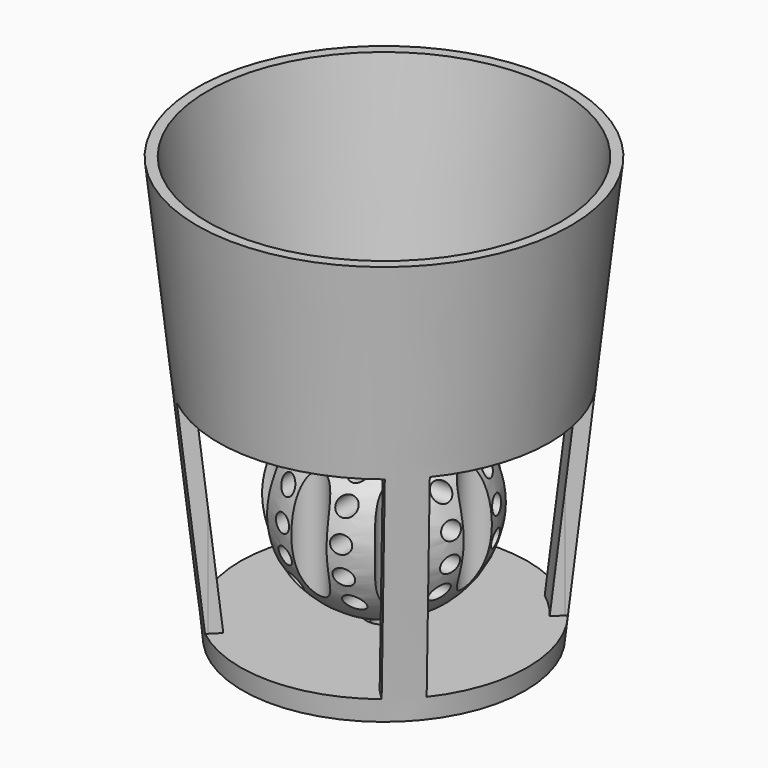
from build123d import *

# Parameters (mm, degrees)
F3_DEPTH      = 29
F4_R          = 2.5
F5_DEPTH      = 2
F5_DEPTH_BACK = 31
F8_R          = 2.5
F9_DEPTH      = 36.6
F10_R         = 1.25
F11_DEPTH     = 15
F12_R         = 1.25
F13_DEPTH     = 15


with BuildPart() as f1:
    # F0 (on Front) → F1 (revolve)
    with BuildSketch(Plane.XZ):
        Polygon((0, 3), (0, 0), (20, 0), (26.4482922192, 60), (25, 60), (22.3132115753, 35), (0, 35), (0, 32), (21.4275722125, 32), (18.3108976399, 3), align=None)
    revolve(axis=Axis((0, 0, 33.5), (0, 0, 1)))

    # F2 (on face) → F3 (cut)
    with BuildSketch(Plane.XY.offset(3)):
        with BuildLine():
            Line((12.2634482474, 15.7989821534), (15.6845353346, 19.2200692405))
            ThreePointArc((15.6845353346, 19.2200692405), (0, 24.8075736474), (-15.6845353346, 19.2200692405))
            Line((-15.6845353346, 19.2200692405), (-12.2634482474, 15.7989821534))
            Line((-12.2634482474, 15.7989821534), (-10.9417147938, 14.4772486998))
            ThreePointArc((-10.9417147938, 14.4772486998), (0, 18.1469516048), (10.9417147938, 14.4772486998))
            Line((10.9417147938, 14.4772486998), (12.2634482474, 15.7989821534))
        make_face()
        with BuildLine():
            Line((19.2200692405, 15.6845353346), (15.7989821534, 12.2634482474))
            Line((15.7989821534, 12.2634482474), (14.4772486998, 10.9417147938))
            ThreePointArc((14.4772486998, 10.9417147938), (18.1469516048, 0), (14.4772486998, -10.9417147938))
            Line((14.4772486998, -10.9417147938), (15.7989821534, -12.2634482474))
            Line((15.7989821534, -12.2634482474), (19.2200692405, -15.6845353346))
            ThreePointArc((19.2200692405, -15.6845353346), (24.8075736474, 0), (19.2200692405, 15.6845353346))
        make_face()
        with BuildLine():
            Line((-14.4772486998, 10.9417147938), (-15.7989821534, 12.2634482474))
            Line((-15.7989821534, 12.2634482474), (-19.2200692405, 15.6845353346))
            ThreePointArc((-19.2200692405, 15.6845353346), (-24.8075736474, 0), (-19.2200692405, -15.6845353346))
            Line((-19.2200692405, -15.6845353346), (-15.7989821534, -12.2634482474))
            Line((-15.7989821534, -12.2634482474), (-14.4772486998, -10.9417147938))
            ThreePointArc((-14.4772486998, -10.9417147938), (-18.1469516048, 0), (-14.4772486998, 10.9417147938))
        make_face()
        with BuildLine():
            Line((15.6845353346, -19.2200692405), (12.2634482474, -15.7989821534))
            Line((12.2634482474, -15.7989821534), (10.9417147938, -14.4772486998))
            ThreePointArc((10.9417147938, -14.4772486998), (0, -18.1469516048), (-10.9417147938, -14.4772486998))
            Line((-10.9417147938, -14.4772486998), (-12.2634482474, -15.7989821534))
            Line((-12.2634482474, -15.7989821534), (-15.6845353346, -19.2200692405))
            ThreePointArc((-15.6845353346, -19.2200692405), (0, -24.8075736474), (15.6845353346, -19.2200692405))
        make_face()
    extrude(amount=F3_DEPTH, mode=Mode.SUBTRACT)

    # F4 (on face) → F5 (cut, two sides)
    with BuildSketch(Plane.XY.offset(3)) as f5_sk:
        Circle(F4_R)
    extrude(amount=-F5_DEPTH, mode=Mode.SUBTRACT)
    extrude(f5_sk.sketch, amount=F5_DEPTH_BACK, mode=Mode.SUBTRACT)


with BuildPart() as f7:
    # F6 (on Front) → F7 (revolve)
    with BuildSketch(Plane.XZ):
        with BuildLine():
            Line((1.5, 33.25), (0, 33.25))
            Line((0, 33.25), (0, 1.75))
            Line((0, 1.75), (1.5, 1.75))
            Line((1.5, 1.75), (1.5, 4.083592135))
            ThreePointArc((1.5, 4.083592135), (13.5, 17.5), (1.5, 30.916407865))
            Line((1.5, 30.916407865), (1.5, 33.25))
        make_face()
    revolve(axis=Axis((0, 0, 17.5), (0, 0, 1)))

    # F8 (on Top) → F9 (cut)
    with BuildSketch(Plane.XY):
        with Locations((-13.5, 0)):
            Circle(F8_R)
        with Locations((-9.545941546, -9.545941546)):
            Circle(F8_R)
        with Locations((0, -13.5)):
            Circle(F8_R)
        with Locations((9.545941546, -9.545941546)):
            Circle(F8_R)
        with Locations((13.5, 0)):
            Circle(F8_R)
        with Locations((9.545941546, 9.545941546)):
            Circle(F8_R)
        with Locations((0, 13.5)):
            Circle(F8_R)
        with Locations((-9.545941546, 9.545941546)):
            Circle(F8_R)
    extrude(amount=F9_DEPTH, mode=Mode.SUBTRACT)

    # F10 (on Right) → F11 (cut, symmetric)
    with BuildSketch(Plane.YZ):
        with Locations((4.0222867392, 27.1767992207)):
            Circle(F10_R)
        with Locations((4.0222867392, 23.5387650006)):
            Circle(F10_R)
        with Locations((4.0222867392, 19.1933350909)):
            Circle(F10_R)
        with Locations((4.0222867392, 14.9489609535)):
            Circle(F10_R)
        with Locations((4.0222867392, 11.0077567747)):
            Circle(F10_R)
        with Locations((-4.0222867392, 19.1933350909)):
            Circle(F10_R)
        with Locations((-4.0222867392, 14.9489609535)):
            Circle(F10_R)
        with Locations((-4.0222867392, 11.0077567747)):
            Circle(F10_R)
        with Locations((-4.0222867392, 23.5387650006)):
            Circle(F10_R)
        with Locations((-4.0222867392, 27.1767992207)):
            Circle(F10_R)
    extrude(amount=F11_DEPTH, both=True, mode=Mode.SUBTRACT)

    # F12 (on Front) → F13 (cut, symmetric)
    with BuildSketch(Plane.XZ):
        with Locations((4.144573817, 26.2041959244)):
            Circle(F12_R)
        with Locations((4.144573817, 22.5661617042)):
            Circle(F12_R)
        with Locations((4.144573817, 18.2207317945)):
            Circle(F12_R)
        with Locations((4.144573817, 13.9763576572)):
            Circle(F12_R)
        with Locations((4.144573817, 10.0351534784)):
            Circle(F12_R)
        with Locations((-4.144573817, 18.2207317945)):
            Circle(F12_R)
        with Locations((-4.144573817, 13.9763576572)):
            Circle(F12_R)
        with Locations((-4.144573817, 10.0351534784)):
            Circle(F12_R)
        with Locations((-4.144573817, 22.5661617042)):
            Circle(F12_R)
        with Locations((-4.144573817, 26.2041959244)):
            Circle(F12_R)
    extrude(amount=F13_DEPTH, both=True, mode=Mode.SUBTRACT)


solid = Compound([f1.part, f7.part])
